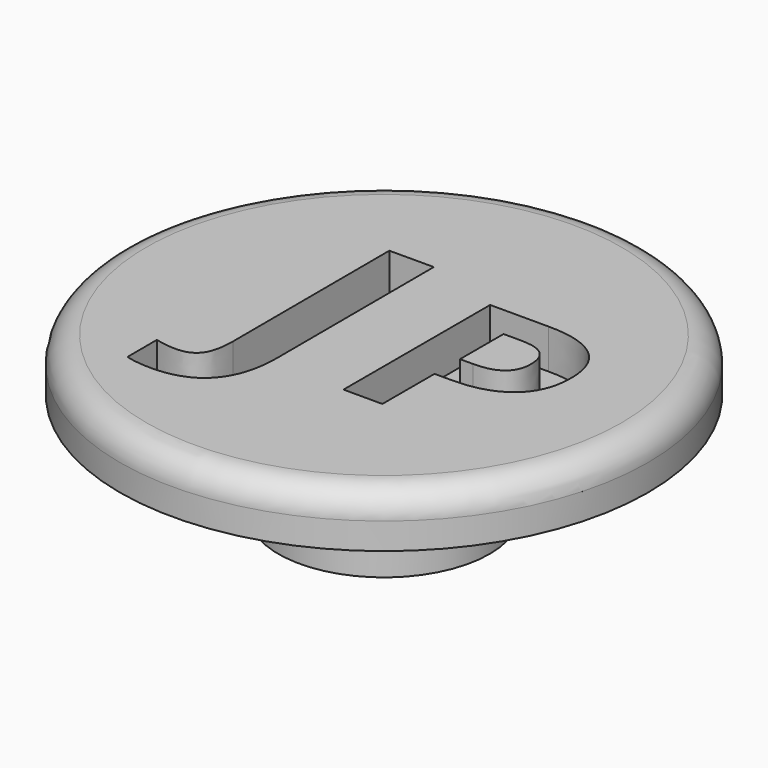
from build123d import *

# Parameters (mm, degrees)
F0_R           = 4
F1_DEPTH       = 6
F0_R_2         = 5
F2_DEPTH       = 2.5
F0_R_3         = 10
F3_DEPTH       = 2
F4_R           = 1
F5_TEXT_SIZE   = 11.1111111111
F5_TEXT_SIZE_2 = 9.7222222222
F6_DEPTH       = 1.5


# Not quite as in the source:
# - Text() gives the source's letters only with a copy of the font that has no kerning and outlines rounded to 1/6400 em; it was checked with that copy


with BuildPart() as f1:
    # F0 (on Top) → F1 (new body)
    with BuildSketch(Plane.XY):
        Circle(F0_R)
    extrude(amount=-F1_DEPTH)

    # F0 (on Top) → F2 (join)
    with BuildSketch(Plane.XY):
        Circle(F0_R_2)
        Circle(F0_R, mode=Mode.SUBTRACT)
    extrude(amount=-F2_DEPTH)

    # F0 (on Top) → F3 (join)
    with BuildSketch(Plane.XY):
        Circle(F0_R_3)
        Circle(F0_R_2, mode=Mode.SUBTRACT)
    extrude(amount=-F3_DEPTH)

    # F4
    f4_edges = [f1.edges().sort_by_distance(p)[0] for p in [
        (-10, 0, 0),
    ]]
    fillet(f4_edges, radius=F4_R)

    # F5 (on Top) → F6 (cut)
    with BuildSketch(Plane.XY):
        with Locations(Location((-4.2256778117, -3.6228192533), (0, 0, 0.160757428))):
            Text('J', F5_TEXT_SIZE, font='Open Sans', font_style=FontStyle.BOLD, text_align=(TextAlign.LEFT, TextAlign.BOTTOM))
        with Locations((0.3761056306, -3.4794011321)):
            Text('P', F5_TEXT_SIZE_2, font='Open Sans', font_style=FontStyle.BOLD, text_align=(TextAlign.LEFT, TextAlign.BOTTOM))
    extrude(amount=-F6_DEPTH, mode=Mode.SUBTRACT)


solid = f1.part
